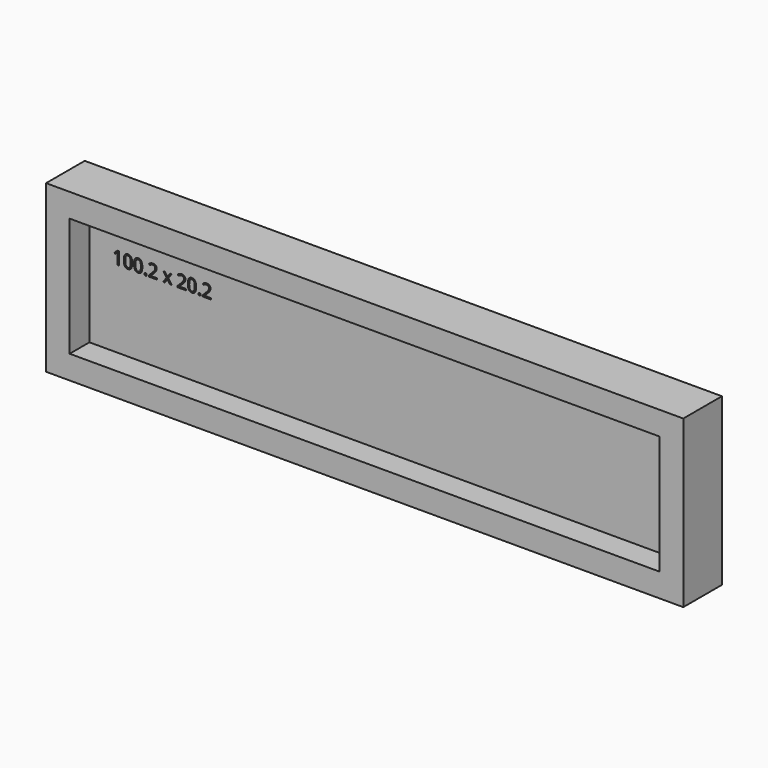
from build123d import *

# Parameters (mm, degrees)
F3_W         = 108.2
F3_H         = 28.2
F4_DEPTH     = 8.2
F5_T         = -4
F6_TEXT_SIZE = 3.0205326362
F7_DEPTH     = 1


# Not quite as in the source:
# - Text() gives the source's letters only with a copy of the font that has no kerning and outlines rounded to 1/6400 em; it was checked with that copy


with BuildPart() as f4:
    # F3 (on Front) → F4 (new body)
    with BuildSketch(Plane.XZ):
        with Locations((54.1, 14.1)):
            Rectangle(F3_W, F3_H)
    extrude(amount=F4_DEPTH)

    # F5
    f5_openings = [f4.faces().sort_by_distance(p)[0] for p in [
        (54.1, -8.2, 14.1),
    ]]
    offset(amount=F5_T, openings=f5_openings)

    # F6 (on face) → F7 (cut)
    with BuildSketch(Plane.XZ.offset(4)):
        with Locations((7.9596647993, 17.0949809253)):
            Text('100.2 x 20.2', F6_TEXT_SIZE, font='Open Sans', text_align=(TextAlign.LEFT, TextAlign.BOTTOM))
    extrude(amount=-F7_DEPTH, mode=Mode.SUBTRACT)


solid = f4.part
